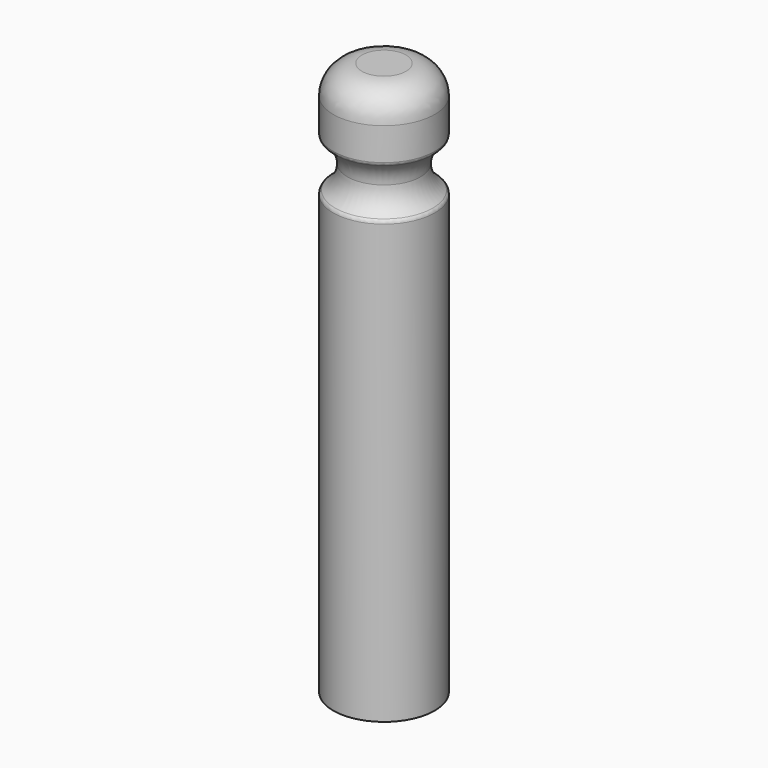
from build123d import *

# Parameters (mm, degrees)
F3_R = 1


# Not quite as in the source:
# - a fillet or chamfer that OpenCascade refuses, or shapes differently, is made with other operations: its cross-section is extruded or revolved along the edge and cut away or added


with BuildPart() as f1:
    # F0 (on Front) → F1 (revolve)
    with BuildSketch(Plane.XZ):
        with BuildLine():
            Line((-11.5, 0), (0, 0))
            Line((0, 0), (0, 125.5))
            Line((0, 125.5), (-11.5, 125.5))
            Line((-11.5, 125.5), (-11.5, 111.1))
            ThreePointArc((-11.5, 111.1), (-11.4175796144, 111.0506064835), (-11.3358983849, 111))
            Line((-11.3358983849, 111), (-8.3, 111))
            Line((-8.3, 111), (-8.3, 105.5))
            Line((-8.3, 105.5), (-8.3, 100))
            Line((-8.3, 100), (-11.3358983849, 100))
            ThreePointArc((-11.3358983849, 100), (-11.4175796144, 99.9493935165), (-11.5, 99.9))
            Line((-11.5, 99.9), (-11.5, 0))
        make_face()
    revolve(axis=Axis((0, 0, 62.75), (0, 0, 1)))

    # F2: fillet of radius 6.5 on 3 edges, made by hand

    # F2_s1 → F2_t2 (revolve, cut)
    with BuildSketch(Plane.XZ):
        with BuildLine():
            ThreePointArc((-11.5, 119), (-9.5961940777, 123.5961940777), (-5, 125.5))
            Line((-5, 125.5), (-11.5, 125.5))
            Line((-11.5, 125.5), (-11.5, 119))
        make_face()
    revolve(axis=Axis((0, 0, 125.5), (0, 0, 1)), mode=Mode.SUBTRACT)

    # F2_s3 → F2_t4 (revolve)
    with BuildSketch(Plane.XZ):
        with BuildLine():
            ThreePointArc((-8.3, 105.5), (-9.1093646884, 108.6411255548), (-11.3358983849, 111))
            Line((-11.3358983849, 111), (-8.3, 111))
            Line((-8.3, 111), (-8.3, 105.5))
        make_face()
    revolve(axis=Axis((0, 0, 111), (0, 0, 1)))

    # F2_s5 → F2_t6 (revolve)
    with BuildSketch(Plane.XZ):
        with BuildLine():
            ThreePointArc((-11.3358983849, 100), (-9.1093646884, 102.3588744452), (-8.3, 105.5))
            Line((-8.3, 105.5), (-8.3, 100))
            Line((-8.3, 100), (-11.3358983849, 100))
        make_face()
    revolve(axis=Axis((0, 0, 100), (0, 0, 1)))

    # F3
    f3_edges = [f1.edges().sort_by_distance(p)[0] for p in [
        (11.5, 0, 111.1),
        (11.5, 0, 99.9),
    ]]
    fillet(f3_edges, radius=F3_R)


solid = f1.part
